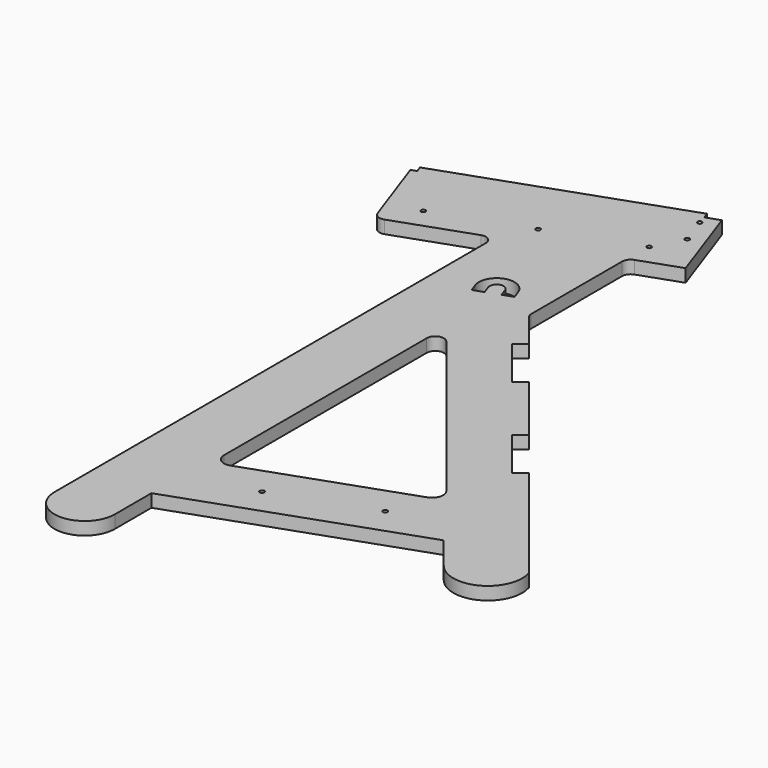
from build123d import *

# Parameters (mm, degrees)
F1_DEPTH = 19.05
F3_DEPTH = 9.525
F5_DEPTH = 9.525
F6_W     = 94.742
F6_H     = 19.05
F6_H_2   = 22.0252738774
F7_DEPTH = 19.558
F8_R     = 3.302
F9_DEPTH = 19.051


# Not quite as in the source:
# - ends of sketch curves that miss each other by under 0.0002 mm in the source are joined
# - a feature names something its author has since deleted; it is built from what else it names
# - the program builds the solid bodies; features that only make, move or delete a surface that nothing else refers to are left out


with BuildPart() as f1:
    # F0 (on Top) → F1 (new body)
    with BuildSketch(Plane.XY):
        with BuildLine():
            Line((727.2677384075, 507.6293858847), (727.2677384075, -289.3185215378))
            ThreePointArc((727.2677384075, -289.3185215378), (771.8616098047, -333.912392935), (816.4554812019, -289.3185215378))
            Line((816.4554812019, -289.3185215378), (816.4554812019, -221.6290421598))
            Line((816.4554812019, -221.6290421598), (1153.5588304871, -102.9697649078))
            Line((1153.5588304871, -102.9697649078), (1192.9737952894, -152.2336658633))
            ThreePointArc((1192.9737952894, -152.2336658633), (1256.5580507142, -165.3785793409), (1281.2649482254, -105.3342998163))
            Line((1281.2649482254, -105.3342998163), (881.6774022659, 394.10141923))
            ThreePointArc((881.6774022659, 394.10141923), (879.6100790274, 397.83144491), (878.8940586752, 402.0355181492))
            Line((878.8940586752, 402.0355181492), (878.8940586752, 569.9420720746))
            ThreePointArc((878.8940586752, 569.9420720746), (881.2296299338, 577.2815963686), (887.3773054254, 581.9215959395))
            Line((887.3773054254, 581.9215959395), (946.5202680448, 602.7397254948))
            Line((946.5202680448, 602.7397254948), (904.3527355464, 722.5349641439))
            Line((904.3527355464, 722.5349641439), (884.020881133, 715.3782178375))
            Line((884.020881133, 715.3782178375), (880.8583161956, 724.3628607361))
            Line((880.8583161956, 724.3628607361), (549.7442765695, 607.8118009104))
            Line((549.7442765695, 607.8118009104), (552.906841507, 598.8271580117))
            Line((552.906841507, 598.8271580117), (544.9670195991, 596.0323666485))
            Line((544.9670195991, 596.0323666485), (582.9177988478, 488.2166518643))
            ThreePointArc((582.9177988478, 488.2166518643), (589.40821497, 480.9809077363), (599.1140759625, 480.4538812492))
            Line((599.1140759625, 480.4538812492), (710.3509851577, 519.6089097496))
            ThreePointArc((710.3509851577, 519.6089097497), (721.9072627016, 517.9938146262), (727.2677384075, 507.6293858847))
        make_face()
        with BuildLine():
            ThreePointArc((844.5095176323, -110.7755588107), (829.4863568252, -108.6759351502), (822.5177384075, -95.2021777863))
            Line((822.5177384075, -95.2021777863), (822.5177384075, 279.3762959499))
            ThreePointArc((822.5177384075, 279.3762959499), (831.0136651683, 291.3602755977), (845.1343948168, 287.3103948691))
            Line((845.1343948168, 287.3103948691), (1078.976974464, -4.9643221252))
            ThreePointArc((1078.976974464, -4.9643221252), (1081.9579117622, -19.8218837855), (1071.5671003568, -30.8520317446))
            Line((1071.5671003568, -30.8520317446), (844.5095176323, -110.7755588107))
        make_face(mode=Mode.SUBTRACT)
        with BuildLine():
            Line((822.1982316908, 418.0308171084), (817.981478441, 430.0103409733))
            ThreePointArc((817.981478441, 430.0103409733), (804.7653209472, 436.3447634256), (798.4309001253, 423.1286012999))
            Line((798.4309001253, 423.1286012999), (802.6476533752, 411.149077435))
            Line((802.6476533752, 411.149077435), (787.6732485441, 405.8781358727))
            Line((787.6732485441, 405.8781358727), (783.4564952942, 417.8576597376))
            ThreePointArc((783.4564952942, 417.8576597376), (799.4943781806, 451.3191657439), (832.9558841868, 435.2812828576))
            Line((832.9558841868, 435.2812828576), (837.1726374367, 423.3017589927))
            Line((837.1726374367, 423.3017589927), (822.1982316908, 418.0308171084))
        make_face(mode=Mode.SUBTRACT)
    extrude(amount=F1_DEPTH)

    # F2 (on face) → F3 (cut)
    with BuildSketch(Plane.XY):
        with BuildLine():
            ThreePointArc((844.1222933391, -166.9052020902), (847.3560158569, -170.6500208272), (852.2954479263, -170.9374917442))
            Line((852.2954479263, -170.9374917442), (1129.8610507564, -72.1108335167))
            ThreePointArc((1129.8610507564, -72.1108335167), (1133.425786756, -68.9382065458), (1133.77435322, -64.1788572139))
            Line((1133.77435322, -64.1788572139), (1131.667577719, -57.6492424267))
            ThreePointArc((1131.667577719, -57.6492424267), (1128.4338552012, -53.9044236898), (1123.4944231318, -53.6169527728))
            Line((1123.4944231318, -53.6169527728), (845.9288203018, -152.4436110002))
            ThreePointArc((845.9288203018, -152.4436110002), (842.3640843021, -155.6162379711), (842.0155178382, -160.3755873031))
            Line((842.0155178382, -160.3755873031), (844.1222933391, -166.9052020902))
        make_face()
    extrude(amount=F3_DEPTH, mode=Mode.SUBTRACT)

    # F4 (on face) → F5 (cut)
    with BuildSketch(Plane.XY):
        Polygon((579.9443241227, 521.366756094), (586.5044770697, 502.9417796404), (921.8787370541, 622.3506942479), (916.3315891482, 637.930524532), (912.1286802343, 636.4340924814), (884.020881133, 715.3782178375), (880.8583161956, 724.3628607361), (862.3802941818, 717.9536434315), (892.7236092325, 632.7308033777), align=None)
    extrude(amount=F5_DEPTH, mode=Mode.SUBTRACT)

    # F6 (on face) → F7 (cut)
    with BuildSketch(Plane(origin=(729.8159568657, 583.9097126711, 0), x_dir=(-0.6247321984, 0.7808390873, 0), z_dir=(0.7808390873, 0.6247321984, 0))):
        with Locations((-357.8801403508, 9.525)):
            Rectangle(F6_W, F6_H)
        with Locations((-584.9891603508, 10.3152221296)):
            Rectangle(F6_W, F6_H_2)
    extrude(amount=-F7_DEPTH, mode=Mode.SUBTRACT)

    # F8 (on face) → F9 (cut, through all)
    with BuildSketch(Plane.XY):
        with BuildLine():
            ThreePointArc((902.3498094673, 663.8992240234), (899.5515171423, 659.5044786379), (904.4975380125, 657.8670707804))
            Line((904.4975380125, 657.8670707804), (902.3498094673, 663.8992240234))
        make_face()
        with BuildLine():
            ThreePointArc((887.5764301967, 705.3920317976), (884.8076232072, 701.0002222812), (889.7289379426, 699.3464555963))
            Line((889.7289379426, 699.3464555963), (887.5764301967, 705.3920317976))
        make_face()
        with BuildLine():
            Line((887.5764301967, 705.3920317976), (889.7289379426, 699.3464555963))
            ThreePointArc((889.7289379426, 699.3464555963), (890.8236579238, 700.5386106967), (891.2203335175, 702.107780571))
            ThreePointArc((891.2203335175, 702.107780571), (890.1290165833, 704.5605513272), (887.5764301967, 705.3920317976))
        make_face()
        with BuildLine():
            Line((902.3498094673, 663.8992240234), (904.4975380125, 657.8670707804))
            ThreePointArc((904.4975380125, 657.8670707804), (905.5745632393, 659.0559185948), (905.9642274527, 660.6120369276))
            ThreePointArc((905.9642274527, 660.6120369276), (904.8838934731, 663.0548639976), (902.3498094673, 663.8992240234))
        make_face()
        with Locations((880.5389518172, 617.9122097817)):
            Circle(F8_R)
        with BuildLine():
            ThreePointArc((623.7483495144, 526.4827509324), (617.3838130375, 524.8132146381), (623.9396392041, 525.3751926427))
            ThreePointArc((623.9396392041, 525.3751926427), (623.8914653707, 525.9371706472), (623.7483495144, 526.4827509324))
        make_face()
        with BuildLine():
            ThreePointArc((756.0284718398, 572.4049919407), (752.1644938352, 575.6588181073), (749.6157615295, 571.2974336509))
            ThreePointArc((749.6157615295, 571.2974336509), (753.2884498444, 569.1511657741), (756.0284718398, 572.4049919407))
        make_face()
        with Locations((1055.4790926394, -88.2571151612)):
            Circle(F8_R)
        with Locations((913.5925848765, -138.7755124943)):
            Circle(F8_R)
    extrude(amount=F9_DEPTH, mode=Mode.SUBTRACT)


solid = f1.part
